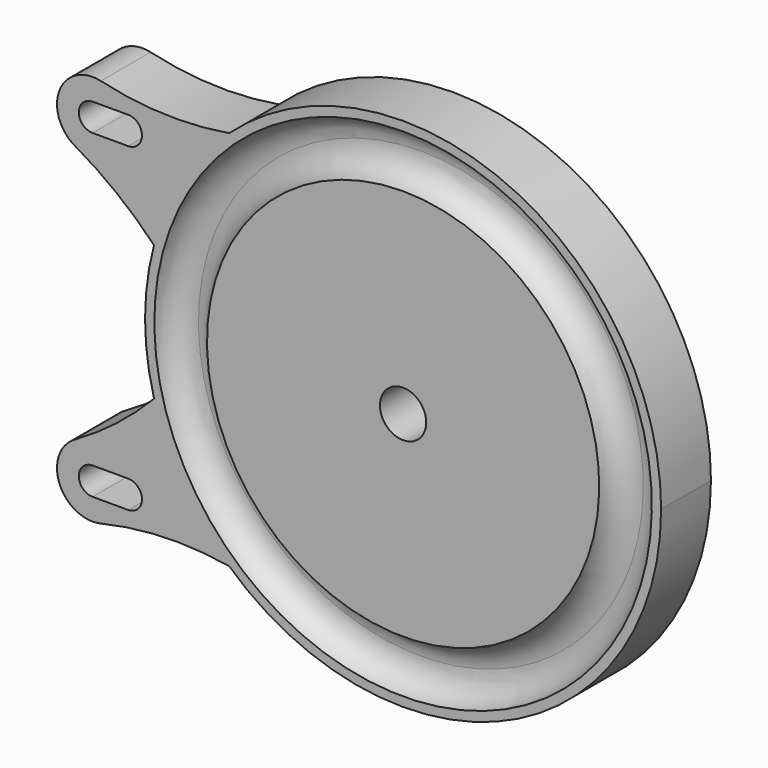
from build123d import *

# Parameters (mm, degrees)
F0_R     = 2.6
F1_DEPTH = 7
F2_R     = 3


# Not quite as in the source:
# - a feature names something its author has since deleted; it is built from what else it names


with BuildPart() as f1:
    # F0 (on Front) → F1 (new body)
    with BuildSketch(Plane.XZ):
        with BuildLine():
            ThreePointArc((-19.5484192549, -21.4210014853), (11.706746807, -26.5320952659), (29, 0))
            ThreePointArc((29, 0), (11.706746807, 26.5320952659), (-19.5484192549, 21.4210014853))
            ThreePointArc((-19.5484192549, 21.4210014853), (-24.7548164348, 15.1062590762), (-27.9895839317, 7.5883589353))
            ThreePointArc((-27.9895839317, 7.5883589353), (-29, 0), (-27.9895839317, -7.5883589353))
            ThreePointArc((-27.9895839317, -7.5883589353), (-24.7548164348, -15.1062590762), (-19.5484192549, -21.4210014853))
        make_face()
        Circle(F0_R, mode=Mode.SUBTRACT)
        with BuildLine():
            ThreePointArc((-27.9895839317, 7.5883589353), (-24.7548164348, 15.1062590762), (-19.5484192549, 21.4210014853))
            ThreePointArc((-19.5484192549, 21.4210014853), (-26.7826801614, 20.9280500488), (-33.9694734381, 21.8911359117))
            ThreePointArc((-33.9694734381, 21.8911359117), (-38.616718272, 19.4692528721), (-36.8782865714, 14.5255440189))
            ThreePointArc((-36.8782865714, 14.5255440189), (-32.1832277785, 11.3781861206), (-27.9895839317, 7.5883589353))
        make_face()
        with BuildLine():
            ThreePointArc((-34.8963290453, 16.45), (-36.4463290453, 18), (-34.8963290453, 19.55))
            Line((-34.8963290453, 19.55), (-30.8963290453, 19.55))
            ThreePointArc((-30.8963290453, 19.55), (-29.3463290453, 18), (-30.8963290453, 16.45))
            Line((-30.8963290453, 16.45), (-34.8963290453, 16.45))
        make_face(mode=Mode.SUBTRACT)
        with BuildLine():
            ThreePointArc((-33.9694734381, -21.8911359117), (-26.7826801614, -20.9280500488), (-19.5484192549, -21.4210014853))
            ThreePointArc((-19.5484192549, -21.4210014853), (-24.7548164348, -15.1062590762), (-27.9895839317, -7.5883589353))
            ThreePointArc((-27.9895839317, -7.5883589353), (-32.1832277785, -11.3781861206), (-36.8782865714, -14.5255440189))
            ThreePointArc((-36.8782865714, -14.5255440189), (-38.616718272, -19.4692528721), (-33.9694734381, -21.8911359117))
        make_face()
        with BuildLine():
            Line((-34.8963290453, -16.45), (-30.8963290453, -16.45))
            ThreePointArc((-30.8963290453, -16.45), (-29.3463290453, -18), (-30.8963290453, -19.55))
            Line((-30.8963290453, -19.55), (-34.8963290453, -19.55))
            ThreePointArc((-34.8963290453, -19.55), (-36.4463290453, -18), (-34.8963290453, -16.45))
        make_face(mode=Mode.SUBTRACT)
    extrude(amount=F1_DEPTH)

    # F2 (on Right) → F3 (revolve, cut)
    with BuildSketch(Plane.YZ):
        with Locations((-7.5, 25)):
            Circle(F2_R)
    revolve(axis=Axis((0, 0, 0), (0, -1, 0)), mode=Mode.SUBTRACT)


solid = f1.part
